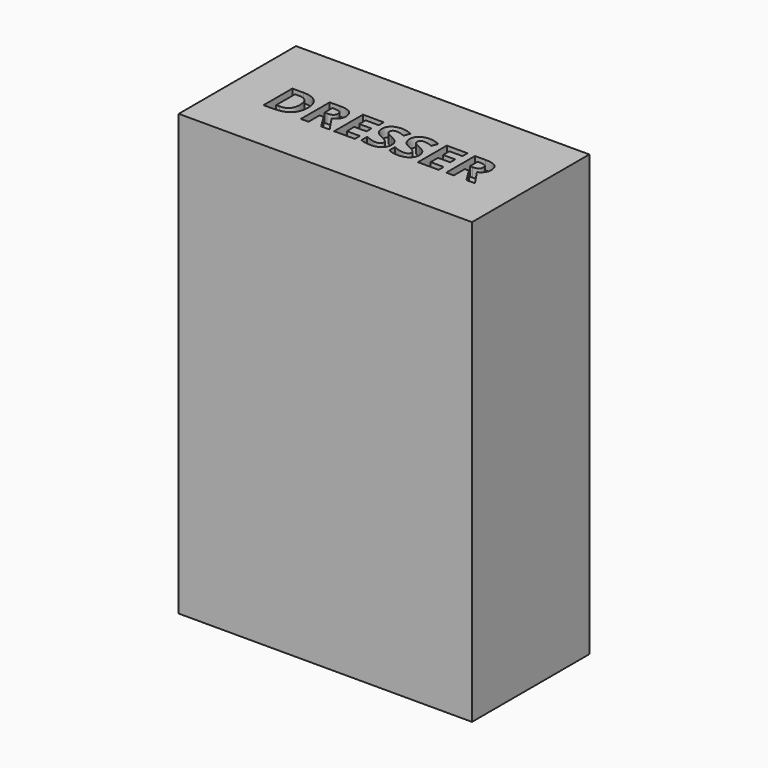
from build123d import *

# Parameters (mm, degrees)
F0_W         = 812.8
F0_H         = 406.4
F1_DEPTH     = 1219.2
F2_TEXT_SIZE = 139.7343662878
F3_DEPTH     = 25.4


# Not quite as in the source:
# - Text() gives the source's letters only with a copy of the font that has no kerning and outlines rounded to 1/6400 em; it was checked with that copy


with BuildPart() as f1:
    # F0 (on Top) → F1 (new body)
    with BuildSketch(Plane.XY):
        with Locations((406.4, 203.2)):
            Rectangle(F0_W, F0_H)
    extrude(amount=F1_DEPTH)

    # F2 (on face) → F3 (cut)
    with BuildSketch(Plane.XY.offset(1219.2)):
        with Locations((105.5198609829, 146.377004683)):
            Text('DRESSER', F2_TEXT_SIZE, font='Open Sans', font_style=FontStyle.BOLD, text_align=(TextAlign.LEFT, TextAlign.BOTTOM))
    extrude(amount=-F3_DEPTH, mode=Mode.SUBTRACT)


solid = f1.part
